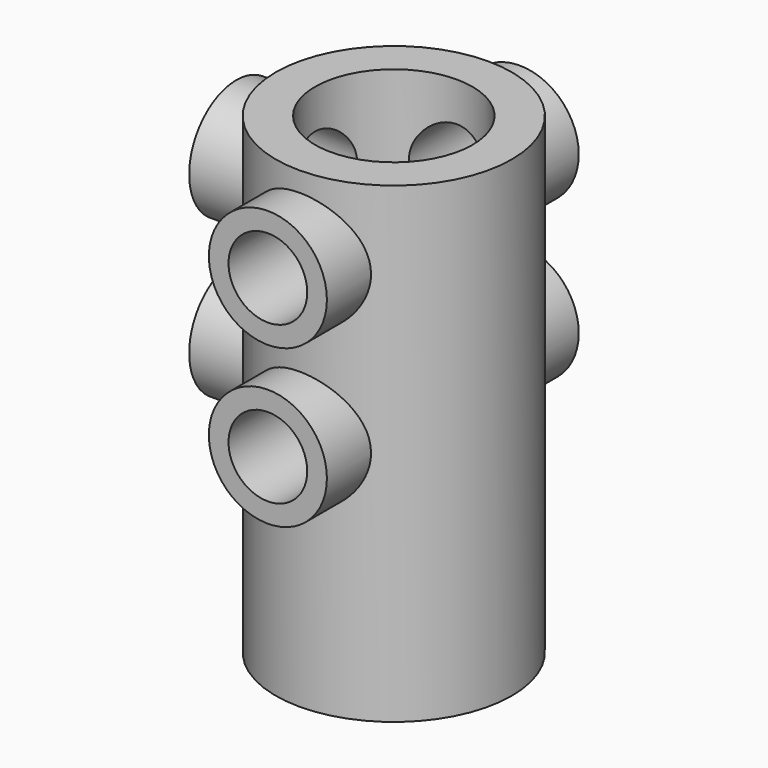
from build123d import *

# Parameters (mm, degrees)
F0_R      = 19.05
F1_DEPTH  = 76.2
F2_R      = 9.525
F3_DEPTH  = 25.4
F4_R      = 9.525
F5_DEPTH  = 25.4
F6_R      = 6.35
F7_DEPTH  = 30.48
F8_R      = 6.35
F9_DEPTH  = 50.8010001
F10_R     = 12.7
F11_DEPTH = 76.2010001


with BuildPart() as f1:
    # F0 (on Top) → F1 (new body)
    with BuildSketch(Plane.XY):
        Circle(F0_R)
    extrude(amount=F1_DEPTH)

    # F2 (on Front) → F3 (join, symmetric)
    with BuildSketch(Plane.XZ):
        with Locations((0, 63.5)):
            Circle(F2_R)
        with Locations((0, 38.1)):
            Circle(F2_R)
    extrude(amount=F3_DEPTH, both=True)

    # F4 (on Right) → F5 (join)
    with BuildSketch(Plane.YZ):
        with Locations((0, 63.5)):
            Circle(F4_R)
        with Locations((0, 38.1)):
            Circle(F4_R)
    extrude(amount=-F5_DEPTH)

    # F6 (on Right) → F7 (cut)
    with BuildSketch(Plane.YZ):
        with Locations((0, 63.5)):
            Circle(F6_R)
        with Locations((0, 38.1)):
            Circle(F6_R)
    extrude(amount=-F7_DEPTH, mode=Mode.SUBTRACT)

    # F8 (on face) → F9 (cut, through all)
    with BuildSketch(Plane.XZ.offset(25.4)):
        with Locations((0, 63.5)):
            Circle(F8_R)
        with Locations((0, 38.1)):
            Circle(F8_R)
    extrude(amount=-F9_DEPTH, mode=Mode.SUBTRACT)

    # F10 (on face) → F11 (cut, through all)
    with BuildSketch(Plane.XY.offset(76.2)):
        Circle(F10_R)
    extrude(amount=-F11_DEPTH, mode=Mode.SUBTRACT)


solid = f1.part
